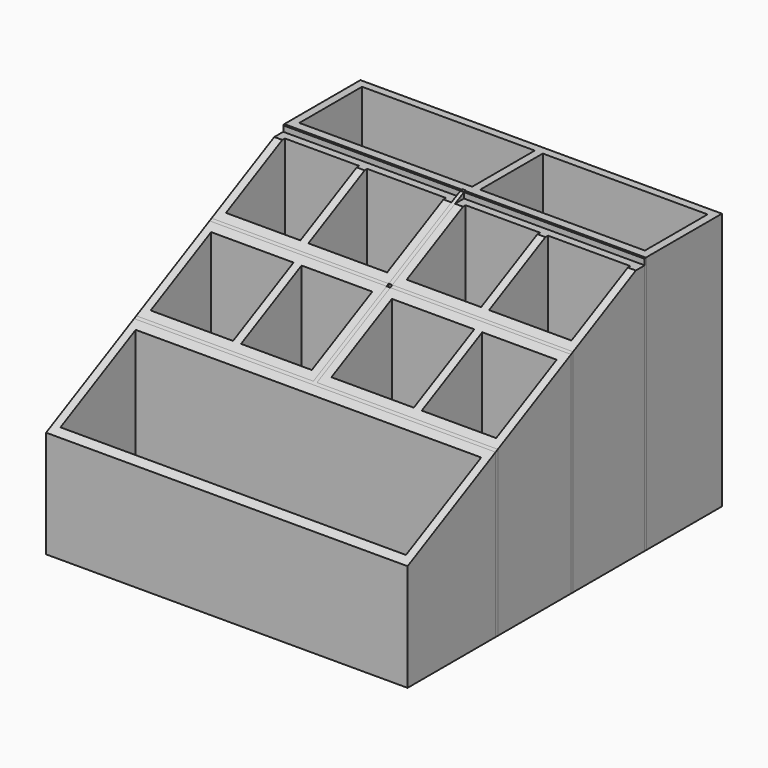
from build123d import *

# Parameters (mm, degrees)
F1_DEPTH  = 82
F2_T      = -2.54
F3_DEPTH  = 82
F4_T      = -2.54
F5_DEPTH  = 52
F6_T      = -2.54
F0_W      = 28.7528
F0_H      = 29.1317389905
F7_DEPTH  = 70
F8_T      = -2.54
F9_DEPTH  = 20
F0_W_2    = 28.7472
F10_DEPTH = 70
F11_T     = -2.54
F12_DEPTH = 20
F13_T     = -2.54
F0_W_3    = 27.5952454776
F14_DEPTH = 70
F15_T     = -2.54
F16_DEPTH = 20
F17_DEPTH = 70
F18_T     = -2.54
F19_DEPTH = 20
F20_T     = -2.54
F0_H_2    = 28.496308485
F21_DEPTH = 80
F22_T     = -2.54
F23_DEPTH = 35
F24_DEPTH = 80
F25_T     = -2.54
F26_DEPTH = 35
F27_DEPTH = 80
F28_T     = -2.54
F29_DEPTH = 35
F30_DEPTH = 80
F31_T     = -2.54
F32_DEPTH = 35
F33_T     = -2.54
F33_2_T   = -2.54
F0_H_3    = 0.8682610095
F0_W_4    = 1.1519545224
F34_DEPTH = 82
F0_H_4    = 0.816094866
F0_H_5    = 0.6875966489
F36_DEPTH = 112.776


# Not quite as in the source:
# - a shell that OpenCascade refuses in one call is made with other operations: the cavity is built on its own and cut out


with BuildPart() as f1:
    # F0 (on Top) → F1 (new body)
    with BuildSketch(Plane.XY):
        Polygon((28.7472, 32.5), (57.5, 32.5), (57.5, 62.5), (0, 62.5), (0, 32.5), align=None)
    extrude(amount=F1_DEPTH)

    # F2
    f2_openings = [f1.faces().sort_by_distance(p)[0] for p in [
        (28.75, 47.5, 82),
    ]]
    offset(amount=F2_T, openings=f2_openings)

    # F0 (on Top) → F3 (join)
    with BuildSketch(Plane.XY):
        Polygon((-57.5, 62.5), (-57.5, 32.5), (-28.7472, 32.5), (-1.1519545224, 32.5), (0, 32.5), (0, 62.5), align=None)
    extrude(amount=F3_DEPTH)

    # F4: a shell. OpenCascade refuses it in one call, so the cavity is built on its own and cut out:
    # the body offset inwards by the wall thickness, plus a prism from it out through each open face.
    f4_core = offset(f1.part, amount=F4_T, kind=Kind.INTERSECTION, mode=Mode.PRIVATE)
    f4_exits = [f4_core.faces().sort_by_distance(p)[0] for p in [
        (-27.48, 47.5, 79.46),
    ]]
    add(f4_core, mode=Mode.SUBTRACT)
    extrude(f4_exits, amount=-F4_T, mode=Mode.SUBTRACT)


with BuildPart() as f5:
    # F0 (on Top) → F5 (new body)
    with BuildSketch(Plane.XY):
        Polygon((-57.5, -62.5), (57.5, -62.5), (57.5, -27.5), (28.7472, -27.5), (0, -27.5), (-28.7472, -27.5), (-57.5, -27.5), align=None)
    extrude(amount=F5_DEPTH)

    # F6
    f6_openings = [f5.faces().sort_by_distance(p)[0] for p in [
        (0, -45, 52),
    ]]
    offset(amount=F6_T, openings=f6_openings)


with BuildPart() as f7:
    # F0 (on Top) → F7 (new body)
    with BuildSketch(Plane.XY):
        with Locations((43.1236, -12.0658694953)):
            Rectangle(F0_W, F0_H)
    extrude(amount=F7_DEPTH)

    # F8
    f8_openings = [f7.faces().sort_by_distance(p)[0] for p in [
        (43.1236, -12.065869, 70),
    ]]
    offset(amount=F8_T, openings=f8_openings)

    # F9 (add): a face of the model
    f9_faces = [f7.faces().sort_by_distance(p)[0] for p in [
        (43.1236, -12.0658694953, 2.54),
    ]]
    extrude(f9_faces, amount=F9_DEPTH)

    # F0 (on Top) → F10 (join)
    with BuildSketch(Plane.XY):
        with Locations((14.3736, -12.0658694953)):
            Rectangle(F0_W_2, F0_H)
    extrude(amount=F10_DEPTH)

    # F11: a shell. OpenCascade refuses it in one call, so the cavity is built on its own and cut out:
    # the body offset inwards by the wall thickness, plus a prism from it out through each open face.
    f11_core = offset(f7.part, amount=F11_T, kind=Kind.INTERSECTION, mode=Mode.PRIVATE)
    f11_exits = [f11_core.faces().sort_by_distance(p)[0] for p in [
        (15.6436, -12.065869, 67.46),
    ]]
    add(f11_core, mode=Mode.SUBTRACT)
    extrude(f11_exits, amount=-F11_T, mode=Mode.SUBTRACT)

    # F12 (add): a face of the model
    f12_faces = [f7.faces().sort_by_distance(p)[0] for p in [
        (28.75, -12.0658694953, 2.54),
    ]]
    extrude(f12_faces, amount=F12_DEPTH)

    # F13: a shell. OpenCascade refuses it in one call, so the cavity is built on its own and cut out:
    # the body offset inwards by the wall thickness, plus a prism from it out through each open face.
    f13_core = offset(f7.part, amount=F13_T, kind=Kind.INTERSECTION, mode=Mode.PRIVATE)
    f13_exits = [f13_core.faces().sort_by_distance(p)[0] for p in [
        (28.75, -12.065869, 2.54),
    ]]
    add(f13_core, mode=Mode.SUBTRACT)
    extrude(f13_exits, amount=-F13_T, mode=Mode.SUBTRACT)


with BuildPart() as f14:
    # F0 (on Top) → F14 (new body)
    with BuildSketch(Plane.XY):
        with Locations((-14.9495772612, -12.0658694953)):
            Rectangle(F0_W_3, F0_H)
    extrude(amount=F14_DEPTH)

    # F15
    f15_openings = [f14.faces().sort_by_distance(p)[0] for p in [
        (-14.949577, -12.065869, 70),
    ]]
    offset(amount=F15_T, openings=f15_openings)

    # F16 (add): a face of the model
    f16_faces = [f14.faces().sort_by_distance(p)[0] for p in [
        (-14.9495772612, -12.0658694953, 2.54),
    ]]
    extrude(f16_faces, amount=F16_DEPTH)

    # F0 (on Top) → F17 (join)
    with BuildSketch(Plane.XY):
        with Locations((-43.1236, -12.0658694953)):
            Rectangle(F0_W, F0_H)
    extrude(amount=F17_DEPTH)

    # F18: a shell. OpenCascade refuses it in one call, so the cavity is built on its own and cut out:
    # the body offset inwards by the wall thickness, plus a prism from it out through each open face.
    f18_core = offset(f14.part, amount=F18_T, kind=Kind.INTERSECTION, mode=Mode.PRIVATE)
    f18_exits = [f18_core.faces().sort_by_distance(p)[0] for p in [
        (-41.8536, -12.065869, 67.46),
    ]]
    add(f18_core, mode=Mode.SUBTRACT)
    extrude(f18_exits, amount=-F18_T, mode=Mode.SUBTRACT)

    # F19 (add): a face of the model
    f19_faces = [f14.faces().sort_by_distance(p)[0] for p in [
        (-29.3259772612, -12.0658694953, 2.54),
    ]]
    extrude(f19_faces, amount=F19_DEPTH)

    # F20: a shell. OpenCascade refuses it in one call, so the cavity is built on its own and cut out:
    # the body offset inwards by the wall thickness, plus a prism from it out through each open face.
    f20_core = offset(f14.part, amount=F20_T, kind=Kind.INTERSECTION, mode=Mode.PRIVATE)
    f20_exits = [f20_core.faces().sort_by_distance(p)[0] for p in [
        (-29.325977, -12.065869, 2.54),
    ]]
    add(f20_core, mode=Mode.SUBTRACT)
    extrude(f20_exits, amount=-F20_T, mode=Mode.SUBTRACT)


with BuildPart() as f21:
    # F0 (on Top) → F21 (new body)
    with BuildSketch(Plane.XY):
        with Locations((-43.1236, 17.5642491085)):
            Rectangle(F0_W, F0_H_2)
    extrude(amount=F21_DEPTH)

    # F22
    f22_openings = [f21.faces().sort_by_distance(p)[0] for p in [
        (-43.1236, 17.564249, 80),
    ]]
    offset(amount=F22_T, openings=f22_openings)

    # F23 (add): a face of the model
    f23_faces = [f21.faces().sort_by_distance(p)[0] for p in [
        (-43.1236, 17.5642491085, 2.54),
    ]]
    extrude(f23_faces, amount=F23_DEPTH)

    # F0 (on Top) → F24 (join)
    with BuildSketch(Plane.XY):
        with Locations((-14.9495772612, 17.5642491085)):
            Rectangle(F0_W_3, F0_H_2)
    extrude(amount=F24_DEPTH)

    # F25: a shell. OpenCascade refuses it in one call, so the cavity is built on its own and cut out:
    # the body offset inwards by the wall thickness, plus a prism from it out through each open face.
    f25_core = offset(f21.part, amount=F25_T, kind=Kind.INTERSECTION, mode=Mode.PRIVATE)
    f25_exits = [f25_core.faces().sort_by_distance(p)[0] for p in [
        (-16.219577, 17.564249, 77.46),
    ]]
    add(f25_core, mode=Mode.SUBTRACT)
    extrude(f25_exits, amount=-F25_T, mode=Mode.SUBTRACT)

    # F26 (add): a face of the model
    f26_faces = [f21.faces().sort_by_distance(p)[0] for p in [
        (-29.3259772612, 17.5642491085, 2.54),
    ]]
    extrude(f26_faces, amount=F26_DEPTH)

    # F33#2: a shell. OpenCascade refuses it in one call, so the cavity is built on its own and cut out:
    # the body offset inwards by the wall thickness, plus a prism from it out through each open face.
    f33_2_core = offset(f21.part, amount=F33_2_T, kind=Kind.INTERSECTION, mode=Mode.PRIVATE)
    f33_2_exits = [f33_2_core.faces().sort_by_distance(p)[0] for p in [
        (-29.325977, 17.564249, 2.54),
    ]]
    add(f33_2_core, mode=Mode.SUBTRACT)
    extrude(f33_2_exits, amount=-F33_2_T, mode=Mode.SUBTRACT)


with BuildPart() as f27:
    # F0 (on Top) → F27 (new body)
    with BuildSketch(Plane.XY):
        with Locations((14.3736, 17.5642491085)):
            Rectangle(F0_W_2, F0_H_2)
    extrude(amount=F27_DEPTH)

    # F28
    f28_openings = [f27.faces().sort_by_distance(p)[0] for p in [
        (14.3736, 17.564249, 80),
    ]]
    offset(amount=F28_T, openings=f28_openings)

    # F29 (add): a face of the model
    f29_faces = [f27.faces().sort_by_distance(p)[0] for p in [
        (14.3736, 17.5642491085, 2.54),
    ]]
    extrude(f29_faces, amount=F29_DEPTH)

    # F0 (on Top) → F30 (join)
    with BuildSketch(Plane.XY):
        with Locations((43.1236, 17.5642491085)):
            Rectangle(F0_W, F0_H_2)
    extrude(amount=F30_DEPTH)

    # F31: a shell. OpenCascade refuses it in one call, so the cavity is built on its own and cut out:
    # the body offset inwards by the wall thickness, plus a prism from it out through each open face.
    f31_core = offset(f27.part, amount=F31_T, kind=Kind.INTERSECTION, mode=Mode.PRIVATE)
    f31_exits = [f31_core.faces().sort_by_distance(p)[0] for p in [
        (41.8536, 17.564249, 77.46),
    ]]
    add(f31_core, mode=Mode.SUBTRACT)
    extrude(f31_exits, amount=-F31_T, mode=Mode.SUBTRACT)

    # F32 (add): a face of the model
    f32_faces = [f27.faces().sort_by_distance(p)[0] for p in [
        (28.75, 17.5642491085, 2.54),
    ]]
    extrude(f32_faces, amount=F32_DEPTH)

    # F33: a shell. OpenCascade refuses it in one call, so the cavity is built on its own and cut out:
    # the body offset inwards by the wall thickness, plus a prism from it out through each open face.
    f33_core = offset(f27.part, amount=F33_T, kind=Kind.INTERSECTION, mode=Mode.PRIVATE)
    f33_exits = [f33_core.faces().sort_by_distance(p)[0] for p in [
        (28.75, 17.564249, 2.54),
    ]]
    add(f33_core, mode=Mode.SUBTRACT)
    extrude(f33_exits, amount=-F33_T, mode=Mode.SUBTRACT)


with BuildPart() as f34:
    # F0 (on Top) → F34 (new body)
    with BuildSketch(Plane.XY):
        Polygon((-28.7472, -26.6317389905), (-28.7472, -27.5), (0, -27.5), (0, -26.6317389905), (-1.1519545224, -26.6317389905), align=None)
        with Locations((-43.1236, -27.0658694953)):
            Rectangle(F0_W, F0_H_3)
        with Locations((43.1236, -27.0658694953)):
            Rectangle(F0_W, F0_H_3)
        with Locations((14.3736, -27.0658694953)):
            Rectangle(F0_W_2, F0_H_3)
        with Locations((-0.5759772612, -12.0658694953)):
            Rectangle(F0_W_4, F0_H)
    extrude(amount=F34_DEPTH)


with BuildPart() as f34b:
    # F0 (on Top) → F34, piece 2 (new body)
    with BuildSketch(Plane.XY):
        with Locations((14.3736, 2.908047433)):
            Rectangle(F0_W_2, F0_H_4)
        with Locations((43.1236, 2.908047433)):
            Rectangle(F0_W, F0_H_4)
    extrude(amount=F34_DEPTH)


with BuildPart() as f34c:
    # F0 (on Top) → F34, piece 3 (new body)
    with BuildSketch(Plane.XY):
        with Locations((-14.9495772612, 2.908047433)):
            Rectangle(F0_W_3, F0_H_4)
        with Locations((-43.1236, 2.908047433)):
            Rectangle(F0_W, F0_H_4)
    extrude(amount=F34_DEPTH)


with BuildPart() as f34d:
    # F0 (on Top) → F34, piece 4 (new body)
    with BuildSketch(Plane.XY):
        with Locations((-43.1236, 32.1562016755)):
            Rectangle(F0_W, F0_H_5)
        with Locations((-14.9495772612, 32.1562016755)):
            Rectangle(F0_W_3, F0_H_5)
    extrude(amount=F34_DEPTH)


with BuildPart() as f34e:
    # F0 (on Top) → F34, piece 5 (new body)
    with BuildSketch(Plane.XY):
        with Locations((-0.5759772612, 17.5642491085)):
            Rectangle(F0_W_4, F0_H_2)
    extrude(amount=F34_DEPTH)


with BuildPart() as f34f:
    # F0 (on Top) → F34, piece 6 (new body)
    with BuildSketch(Plane.XY):
        with Locations((14.3736, 32.1562016755)):
            Rectangle(F0_W_2, F0_H_5)
        with Locations((43.1236, 32.1562016755)):
            Rectangle(F0_W, F0_H_5)
    extrude(amount=F34_DEPTH)


with BuildPart() as f36_tool:
    # F35 (on Right) → F36 (new body, symmetric)
    with BuildSketch(Plane.YZ):
        Polygon((-62.7673566341, 33.945877105), (32.7664129436, 82.2843536735), (33.6038582027, 108.728043735), (-62.7673566341, 108.728043735), align=None)
    extrude(amount=F36_DEPTH, both=True)


with BuildPart() as f5_1:
    add(f5.part)

    # F36: cut by f36_tool
    add(f36_tool.part, mode=Mode.SUBTRACT)


with BuildPart() as f7_1:
    add(f7.part)

    # F36: cut by f36_tool
    add(f36_tool.part, mode=Mode.SUBTRACT)


with BuildPart() as f14_1:
    add(f14.part)

    # F36: cut by f36_tool
    add(f36_tool.part, mode=Mode.SUBTRACT)


with BuildPart() as f21_1:
    add(f21.part)

    # F36: cut by f36_tool
    add(f36_tool.part, mode=Mode.SUBTRACT)


with BuildPart() as f27_1:
    add(f27.part)

    # F36: cut by f36_tool
    add(f36_tool.part, mode=Mode.SUBTRACT)


with BuildPart() as f34_1:
    add(f34.part)

    # F36: cut by f36_tool
    add(f36_tool.part, mode=Mode.SUBTRACT)


with BuildPart() as f34b_1:
    add(f34b.part)

    # F36: cut by f36_tool
    add(f36_tool.part, mode=Mode.SUBTRACT)


with BuildPart() as f34c_1:
    add(f34c.part)

    # F36: cut by f36_tool
    add(f36_tool.part, mode=Mode.SUBTRACT)


with BuildPart() as f34d_1:
    add(f34d.part)

    # F36: cut by f36_tool
    add(f36_tool.part, mode=Mode.SUBTRACT)


with BuildPart() as f34e_1:
    add(f34e.part)

    # F36: cut by f36_tool
    add(f36_tool.part, mode=Mode.SUBTRACT)


with BuildPart() as f34f_1:
    add(f34f.part)

    # F36: cut by f36_tool
    add(f36_tool.part, mode=Mode.SUBTRACT)


solid = Compound([f1.part, f5_1.part, f7_1.part, f14_1.part, f21_1.part, f27_1.part, f34_1.part, f34b_1.part, f34c_1.part, f34d_1.part, f34e_1.part, f34f_1.part])
